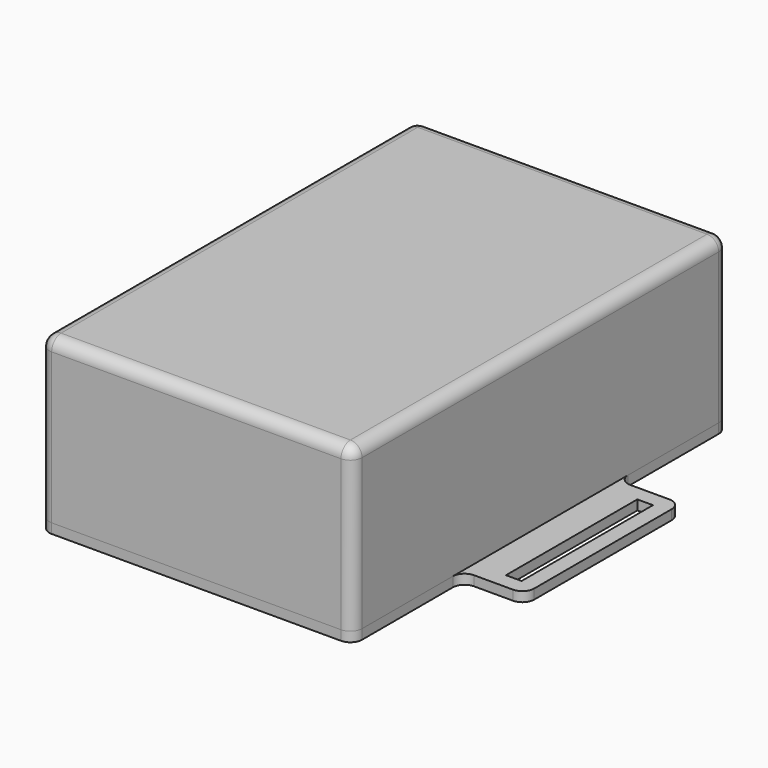
from build123d import *

# Parameters (mm, degrees)
F4_DEPTH  = 1.25
F3_R      = 1.5
F5_DEPTH  = 2
F7_W      = 40
F7_H      = 60
F7_W_2    = 37
F7_H_2    = 57
F8_DEPTH  = 20
F9_W      = 40
F9_H      = 60
F9_W_2    = 37
F9_H_2    = 57
F10_DEPTH = 0.75
F11_R     = 1.5
F11_2_R   = 1.5


with BuildPart() as f4:
    # F3 (on Top) → F4 (new body)
    with BuildSketch(Plane.XY):
        Polygon((-20, 0), (-20, 12.5), (-28, 12.5), (-28, 0), (-28, -12.5), (-20, -12.5), align=None)
        Polygon((-24, 10.5), (-24, 0), (-24, -10.5), (-26, -10.5), (-26, 0), (-26, 10.5), align=None, mode=Mode.SUBTRACT)
        Polygon((28, 12.5), (20, 12.5), (20, 0), (20, -12.5), (28, -12.5), (28, 0), align=None)
        Polygon((24, -10.5), (24, 0), (24, 10.5), (26, 10.5), (26, 0), (26, -10.5), align=None, mode=Mode.SUBTRACT)
        Polygon((20, 30), (0, 30), (-20, 30), (-20, 12.5), (-20, 0), (-20, -12.5), (-20, -30), (0, -30), (20, -30), (20, -12.5), (20, 0), (20, 12.5), align=None)
        Polygon((-18, 28), (0, 28), (18, 28), (18, 0), (18, -28), (0, -28), (-18, -28), (-18, 0), align=None, mode=Mode.SUBTRACT)
    extrude(amount=F4_DEPTH)

    # F3 (on Top) → F5 (join)
    with BuildSketch(Plane.XY):
        Polygon((18, 28), (0, 28), (-18, 28), (-18, 0), (-18, -28), (0, -28), (18, -28), (18, 0), align=None)
        Circle(F3_R, mode=Mode.SUBTRACT)
    extrude(amount=F5_DEPTH)

    # F11#2
    f11_2_edges = [f4.edges().sort_by_distance(p)[0] for p in [
        (-20, 30, 0.625),
        (20, 30, 0.625),
        (-20, -30, 0.625),
        (-28, -12.5, 0.625),
        (-28, 12.5, 0.625),
        (-20, 12.5, 0.625),
        (-20, -12.5, 0.625),
        (20, -30, 0.625),
        (28, -12.5, 0.625),
        (20, -12.5, 0.625),
        (28, 12.5, 0.625),
        (20, 12.5, 0.625),
    ]]
    fillet(f11_2_edges, radius=F11_2_R)


with BuildPart() as f8:
    # F7 (on offset) → F8 (new body)
    with BuildSketch(Plane.XY.offset(1.25)):
        Rectangle(F7_W, F7_H)
        Rectangle(F7_W_2, F7_H_2, mode=Mode.SUBTRACT)
    extrude(amount=F8_DEPTH)

    # F9 (on face) → F10 (join)
    with BuildSketch(Plane.XY.offset(21.25)):
        Rectangle(F9_W, F9_H)
        Rectangle(F9_W_2, F9_H_2, mode=Mode.SUBTRACT)
        Rectangle(F9_W_2, F9_H_2)
    extrude(amount=F10_DEPTH)

    # F11
    f11_edges = [f8.edges().sort_by_distance(p)[0] for p in [
        (0, -30, 22),
        (-20, 0, 22),
        (0, 30, 22),
        (20, 0, 22),
        (20, -30, 11.625),
        (20, 30, 11.625),
        (-20, -30, 11.625),
        (-20, 30, 11.625),
    ]]
    fillet(f11_edges, radius=F11_R)


solid = Compound([f4.part, f8.part])
